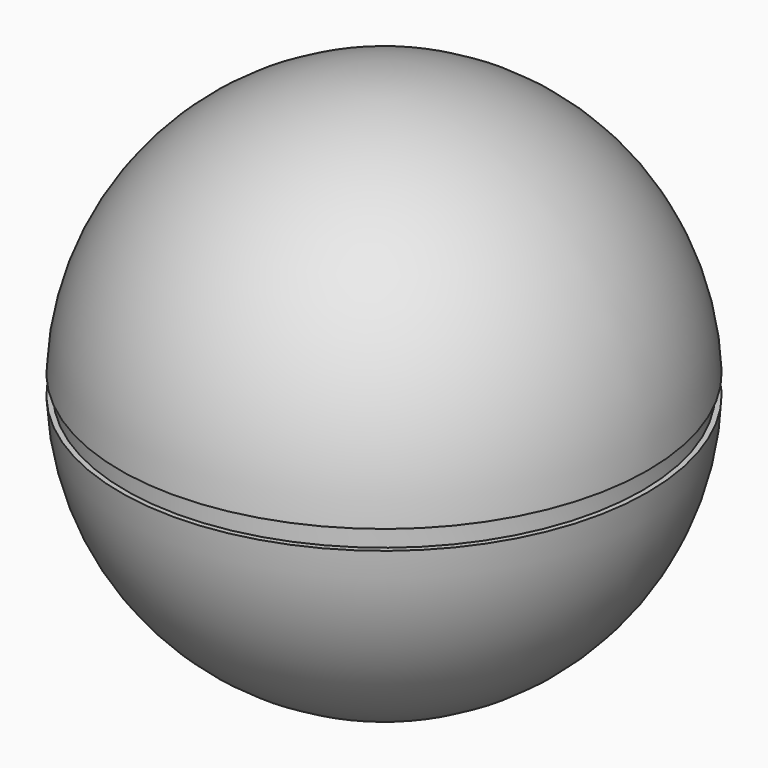
from build123d import *


# Not quite as in the source:
# - the program builds the solid bodies; features that only make, move or delete a surface that nothing else refers to are left out


with BuildPart() as f1:
    # F0 (on Front) → F1 (revolve)
    with BuildSketch(Plane.XZ):
        with BuildLine():
            Line((0, 34.7669126303), (0, -34.7669126303))
            ThreePointArc((0, -34.7669126303), (24.1307297321, -25.0289052186), (34.7437089822, -1.27))
            Line((34.7437089822, -1.27), (34.0511506106, -1.27))
            Line((34.0511506106, -1.27), (34.0511506106, 0))
            Line((34.0511506106, 0), (34.0511506106, 1.27))
            Line((34.0511506106, 1.27), (34.7437089822, 1.27))
            ThreePointArc((34.7437089822, 1.27), (24.1307297321, 25.0289052186), (0, 34.7669126303))
        make_face()
    revolve(axis=Axis((0, 0, 0), (0, 0, -1)))


solid = f1.part
